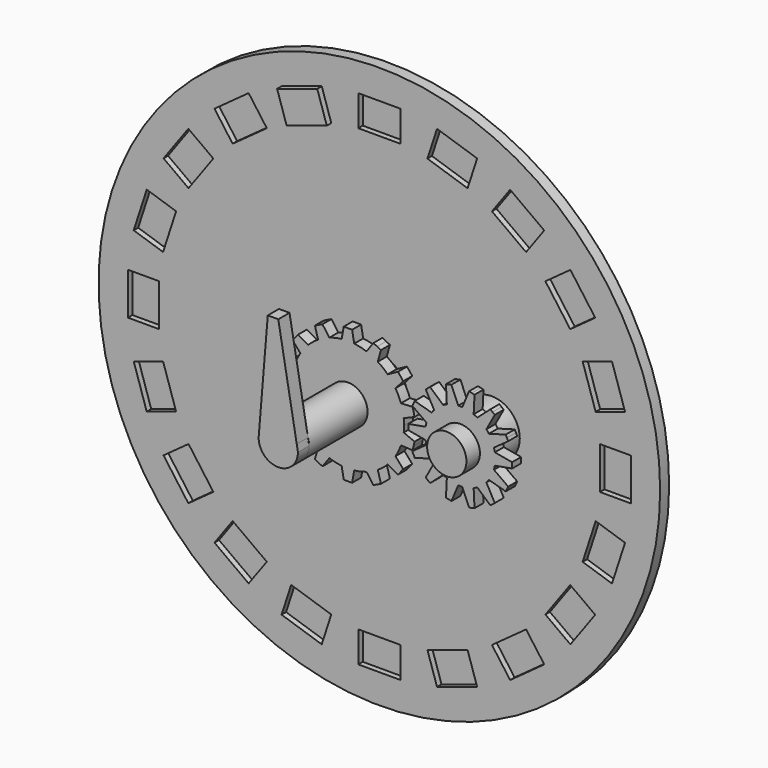
from build123d import *

# Parameters (mm, degrees)
F0_R      = 100
F1_DEPTH  = 4
F2_R      = 10
F2_R_2    = 7
F3_DEPTH  = 10
F4_DEPTH  = 40
F5_DEPTH  = 20
F7_DEPTH  = 4
F9_DEPTH  = 4
F10_W     = 15.0254992768
F10_H     = 11
F10_W_2   = 11
F10_H_2   = 15.0254992768
F11_DEPTH = 2
F12_DEPTH = 4
F14_DEPTH = 5


with BuildPart() as f1:
    # F0 (on Front) → F1 (new body)
    with BuildSketch(Plane.XZ):
        Circle(F0_R)
    extrude(amount=F1_DEPTH)

    # F2 (on face) → F3 (join)
    with BuildSketch(Plane.XZ.offset(4)):
        Circle(F2_R)
        Circle(F2_R_2, mode=Mode.SUBTRACT)
        with Locations((40, 0)):
            Circle(F2_R)
        with Locations((40, 0)):
            Circle(F2_R_2, mode=Mode.SUBTRACT)
    extrude(amount=F3_DEPTH)


with BuildPart() as f4:
    # F4 (new): a face of the model
    f4_faces = [f1.part.faces().sort_by_distance(p)[0] for p in [
        (0, -4, 0),
    ]]
    extrude(f4_faces, amount=F4_DEPTH)

    # F6 (on face) → F7 (join)
    with BuildSketch(Plane.XZ.offset(14)):
        with BuildLine():
            ThreePointArc((19.8728833209, -2.2513348298), (19.9681955421, -1.1274603281), (20, 0))
            ThreePointArc((20, 0), (19.9681955421, 1.1274603281), (19.8728833209, 2.2513348298))
            ThreePointArc((19.8728833209, 2.2513348298), (19.4985582436, 4.4504186791), (18.8816667615, 6.5941383294))
            ThreePointArc((18.8816667615, 6.5941383294), (18.019377358, 8.6776747824), (16.9280316136, 10.6509035152))
            ThreePointArc((16.9280316136, 10.6509035152), (15.6366296494, 12.4697960372), (14.1507045316, 14.1335615207))
            ThreePointArc((14.1507045316, 14.1335615207), (12.4697960372, 15.6366296494), (10.6303756366, 16.9409301346))
            ThreePointArc((10.6303756366, 16.9409301346), (8.6776747824, 18.019377358), (6.6170217222, 18.8736595161))
            ThreePointArc((6.6170217222, 18.8736595161), (4.4504186791, 19.4985582436), (2.2272433917, 19.875597774))
            ThreePointArc((2.2272433917, 19.875597774), (0, 20), (-2.2272433917, 19.875597774))
            ThreePointArc((-2.2272433917, 19.875597774), (-4.4504186791, 19.4985582436), (-6.6170217222, 18.8736595161))
            ThreePointArc((-6.6170217222, 18.8736595161), (-8.6776747824, 18.019377358), (-10.6303756366, 16.9409301346))
            ThreePointArc((-10.6303756366, 16.9409301346), (-12.4697960372, 15.6366296494), (-14.1507045316, 14.1335615207))
            ThreePointArc((-14.1507045316, 14.1335615207), (-15.6366296494, 12.4697960372), (-16.9280316136, 10.6509035152))
            ThreePointArc((-16.9280316136, 10.6509035152), (-18.019377358, 8.6776747824), (-18.8816667615, 6.5941383294))
            ThreePointArc((-18.8816667615, 6.5941383294), (-19.4985582436, 4.4504186791), (-19.8728833209, 2.2513348298))
            ThreePointArc((-19.8728833209, 2.2513348298), (-20, 0), (-19.8728833209, -2.2513348298))
            ThreePointArc((-19.8728833209, -2.2513348298), (-19.4985582436, -4.4504186791), (-18.8816667615, -6.5941383294))
            ThreePointArc((-18.8816667615, -6.5941383294), (-18.019377358, -8.6776747824), (-16.9280316136, -10.6509035152))
            ThreePointArc((-16.9280316136, -10.6509035152), (-15.6366296494, -12.4697960372), (-14.1507045316, -14.1335615207))
            ThreePointArc((-14.1507045316, -14.1335615207), (-12.4697960372, -15.6366296494), (-10.6303756366, -16.9409301346))
            ThreePointArc((-10.6303756366, -16.9409301346), (-8.6776747824, -18.019377358), (-6.6170217222, -18.8736595161))
            ThreePointArc((-6.6170217222, -18.8736595161), (-4.4504186791, -19.4985582436), (-2.2272433917, -19.875597774))
            ThreePointArc((-2.2272433917, -19.875597774), (0, -20), (2.2272433917, -19.875597774))
            ThreePointArc((2.2272433917, -19.875597774), (4.4504186791, -19.4985582436), (6.6170217222, -18.8736595161))
            ThreePointArc((6.6170217222, -18.8736595161), (8.6776747824, -18.019377358), (10.6303756366, -16.9409301346))
            ThreePointArc((10.6303756366, -16.9409301346), (12.4697960372, -15.6366296494), (14.1507045316, -14.1335615207))
            ThreePointArc((14.1507045316, -14.1335615207), (15.6366296494, -12.4697960372), (16.9280316136, -10.6509035152))
            ThreePointArc((16.9280316136, -10.6509035152), (18.019377358, -8.6776747824), (18.8816667615, -6.5941383294))
            ThreePointArc((18.8816667615, -6.5941383294), (19.4985582436, -4.4504186791), (19.8728833209, -2.2513348298))
        make_face()
        with BuildLine():
            ThreePointArc((18.8816667615, 6.5941383294), (19.4985582436, 4.4504186791), (19.8728833209, 2.2513348298))
            Line((19.8728833209, 2.2513348298), (23.7320512933, 3.8781105467))
            Line((23.7320512933, 3.8781105467), (23.3982698924, 5.340502415))
            Line((23.3982698924, 5.340502415), (23.0644884914, 6.8028942832))
            Line((23.0644884914, 6.8028942832), (18.8816667615, 6.5941383294))
        make_face()
        with BuildLine():
            Line((23.7320512933, -3.8781105467), (19.8728833209, -2.2513348298))
            ThreePointArc((19.8728833209, -2.2513348298), (19.4985582436, -4.4504186791), (18.8816667615, -6.5941383294))
            Line((18.8816667615, -6.5941383294), (23.0644884914, -6.8028942832))
            Line((23.0644884914, -6.8028942832), (23.3982698924, -5.340502415))
            Line((23.3982698924, -5.340502415), (23.7320512933, -3.8781105467))
        make_face()
        with BuildLine():
            ThreePointArc((14.1507045316, 14.1335615207), (15.6366296494, 12.4697960372), (16.9280316136, 10.6509035152))
            Line((16.9280316136, 10.6509035152), (19.699190282, 13.7910080209))
            Line((19.699190282, 13.7910080209), (18.7639555792, 14.9637552446))
            Line((18.7639555792, 14.9637552446), (17.8287208764, 16.1365024683))
            Line((17.8287208764, 16.1365024683), (14.1507045316, 14.1335615207))
        make_face()
        with BuildLine():
            Line((19.699190282, -13.7910080209), (16.9280316136, -10.6509035152))
            ThreePointArc((16.9280316136, -10.6509035152), (15.6366296494, -12.4697960372), (14.1507045316, -14.1335615207))
            Line((14.1507045316, -14.1335615207), (17.8287208764, -16.1365024683))
            Line((17.8287208764, -16.1365024683), (18.7639555792, -14.9637552446))
            Line((18.7639555792, -14.9637552446), (19.699190282, -13.7910080209))
        make_face()
        with BuildLine():
            ThreePointArc((6.6170217222, 18.8736595161), (8.6776747824, 18.019377358), (10.6303756366, 16.9409301346))
            Line((10.6303756366, 16.9409301346), (11.7646630407, 20.972427221))
            Line((11.7646630407, 20.972427221), (10.4132097388, 21.6232528297))
            Line((10.4132097388, 21.6232528297), (9.061756437, 22.2740784383))
            Line((9.061756437, 22.2740784383), (6.6170217222, 18.8736595161))
        make_face()
        with BuildLine():
            Line((11.7646630407, -20.972427221), (10.6303756366, -16.9409301346))
            ThreePointArc((10.6303756366, -16.9409301346), (8.6776747824, -18.019377358), (6.6170217222, -18.8736595161))
            Line((6.6170217222, -18.8736595161), (9.061756437, -22.2740784383))
            Line((9.061756437, -22.2740784383), (10.4132097388, -21.6232528297))
            Line((10.4132097388, -21.6232528297), (11.7646630407, -20.972427221))
        make_face()
        with BuildLine():
            ThreePointArc((-2.2272433917, 19.875597774), (0, 20), (2.2272433917, 19.875597774))
            Line((2.2272433917, 19.875597774), (1.5, 24))
            Line((1.5, 24), (0, 24))
            Line((0, 24), (-1.5, 24))
            Line((-1.5, 24), (-2.2272433917, 19.875597774))
        make_face()
        with BuildLine():
            Line((1.5, -24), (2.2272433917, -19.875597774))
            ThreePointArc((2.2272433917, -19.875597774), (0, -20), (-2.2272433917, -19.875597774))
            Line((-2.2272433917, -19.875597774), (-1.5, -24))
            Line((-1.5, -24), (0, -24))
            Line((0, -24), (1.5, -24))
        make_face()
        with BuildLine():
            ThreePointArc((-10.6303756366, 16.9409301346), (-8.6776747824, 18.019377358), (-6.6170217222, 18.8736595161))
            Line((-6.6170217222, 18.8736595161), (-9.061756437, 22.2740784383))
            Line((-9.061756437, 22.2740784383), (-10.4132097388, 21.6232528297))
            Line((-10.4132097388, 21.6232528297), (-11.7646630407, 20.972427221))
            Line((-11.7646630407, 20.972427221), (-10.6303756366, 16.9409301346))
        make_face()
        with BuildLine():
            Line((-9.061756437, -22.2740784383), (-6.6170217222, -18.8736595161))
            ThreePointArc((-6.6170217222, -18.8736595161), (-8.6776747824, -18.019377358), (-10.6303756366, -16.9409301346))
            Line((-10.6303756366, -16.9409301346), (-11.7646630407, -20.972427221))
            Line((-11.7646630407, -20.972427221), (-10.4132097388, -21.6232528297))
            Line((-10.4132097388, -21.6232528297), (-9.061756437, -22.2740784383))
        make_face()
        with BuildLine():
            ThreePointArc((-16.9280316136, 10.6509035152), (-15.6366296494, 12.4697960372), (-14.1507045316, 14.1335615207))
            Line((-14.1507045316, 14.1335615207), (-17.8287208764, 16.1365024683))
            Line((-17.8287208764, 16.1365024683), (-18.7639555792, 14.9637552446))
            Line((-18.7639555792, 14.9637552446), (-19.699190282, 13.7910080209))
            Line((-19.699190282, 13.7910080209), (-16.9280316136, 10.6509035152))
        make_face()
        with BuildLine():
            Line((-17.8287208764, -16.1365024683), (-14.1507045316, -14.1335615207))
            ThreePointArc((-14.1507045316, -14.1335615207), (-15.6366296494, -12.4697960372), (-16.9280316136, -10.6509035152))
            Line((-16.9280316136, -10.6509035152), (-19.699190282, -13.7910080209))
            Line((-19.699190282, -13.7910080209), (-18.7639555792, -14.9637552446))
            Line((-18.7639555792, -14.9637552446), (-17.8287208764, -16.1365024683))
        make_face()
        with BuildLine():
            ThreePointArc((-19.8728833209, 2.2513348298), (-19.4985582436, 4.4504186791), (-18.8816667615, 6.5941383294))
            Line((-18.8816667615, 6.5941383294), (-23.0644884914, 6.8028942832))
            Line((-23.0644884914, 6.8028942832), (-23.3982698924, 5.340502415))
            Line((-23.3982698924, 5.340502415), (-23.7320512933, 3.8781105467))
            Line((-23.7320512933, 3.8781105467), (-19.8728833209, 2.2513348298))
        make_face()
        with BuildLine():
            Line((-23.0644884914, -6.8028942832), (-18.8816667615, -6.5941383294))
            ThreePointArc((-18.8816667615, -6.5941383294), (-19.4985582436, -4.4504186791), (-19.8728833209, -2.2513348298))
            Line((-19.8728833209, -2.2513348298), (-23.7320512933, -3.8781105467))
            Line((-23.7320512933, -3.8781105467), (-23.3982698924, -5.340502415))
            Line((-23.3982698924, -5.340502415), (-23.0644884914, -6.8028942832))
        make_face()
    extrude(amount=F7_DEPTH)

    # F13 (on face) → F14 (join)
    with BuildSketch(Plane.XZ.offset(44)):
        with BuildLine():
            Line((-6.905075168, 1.1488850788), (-7, 0))
            ThreePointArc((-7, 0), (0, -7), (7, 0))
            Line((7, 0), (6.57125, 2.4121926618))
            ThreePointArc((6.57125, 2.4121926618), (-0.653334771, 6.9694442875), (-6.905075168, 1.1488850788))
        make_face()
        with BuildLine():
            Line((-3.7460629491, 39.382737335), (-6.905075168, 1.1488850788))
            ThreePointArc((-6.905075168, 1.1488850788), (-0.653334771, 6.9694442875), (6.57125, 2.4121926618))
            Line((6.57125, 2.4121926618), (0, 39.382737335))
            Line((0, 39.382737335), (-3.7460629491, 39.382737335))
        make_face()
    extrude(amount=F14_DEPTH)


with BuildPart() as f5:
    # F5 (new): a face of the model
    f5_faces = [f1.part.faces().sort_by_distance(p)[0] for p in [
        (40, -4, 0),
    ]]
    extrude(f5_faces, amount=F5_DEPTH)

    # F8 (on face) → F9 (join)
    with BuildSketch(Plane.XZ.offset(14)):
        with BuildLine():
            ThreePointArc((52.3250464347, -2.0840418379), (52.4561848179, -1.0456862737), (52.5, 0))
            ThreePointArc((52.5, 0), (52.4561848179, 1.0456862737), (52.3250464347, 2.0840418379))
            ThreePointArc((52.3250464347, 2.0840418379), (52.1865989023, 2.7815116745), (52.0087149982, 3.4699804165))
            ThreePointArc((52.0087149982, 3.4699804165), (51.2621108488, 5.423546739), (50.200251268, 7.2252940473))
            ThreePointArc((50.200251268, 7.2252940473), (49.7728935309, 7.7936225232), (49.3139102792, 8.3367304929))
            ThreePointArc((49.3139102792, 8.3367304929), (47.7936225232, 9.7728935309), (46.0551712398, 10.9354881581))
            ThreePointArc((46.0551712398, 10.9354881581), (45.423546739, 11.2621108488), (44.7743714017, 11.552288852))
            ThreePointArc((44.7743714017, 11.552288852), (42.7815116745, 12.1865989023), (40.7107902857, 12.4797747243))
            ThreePointArc((40.7107902857, 12.4797747243), (40, 12.5), (39.2892097143, 12.4797747243))
            ThreePointArc((39.2892097143, 12.4797747243), (37.2184883255, 12.1865989023), (35.2256285983, 11.552288852))
            ThreePointArc((35.2256285983, 11.552288852), (34.576453261, 11.2621108488), (33.9448287602, 10.9354881581))
            ThreePointArc((33.9448287602, 10.9354881581), (32.2063774768, 9.7728935309), (30.6860897208, 8.3367304929))
            ThreePointArc((30.6860897208, 8.3367304929), (30.2271064691, 7.7936225232), (29.799748732, 7.2252940473))
            ThreePointArc((29.799748732, 7.2252940473), (28.7378891512, 5.423546739), (27.9912850018, 3.4699804165))
            ThreePointArc((27.9912850018, 3.4699804165), (27.8134010977, 2.7815116745), (27.6749535653, 2.0840418379))
            ThreePointArc((27.6749535653, 2.0840418379), (27.5, 0), (27.6749535653, -2.0840418379))
            ThreePointArc((27.6749535653, -2.0840418379), (27.8134010977, -2.7815116745), (27.9912850018, -3.4699804165))
            ThreePointArc((27.9912850018, -3.4699804165), (28.7378891512, -5.423546739), (29.799748732, -7.2252940473))
            ThreePointArc((29.799748732, -7.2252940473), (30.2271064691, -7.7936225232), (30.6860897208, -8.3367304929))
            ThreePointArc((30.6860897208, -8.3367304929), (32.2063774768, -9.7728935309), (33.9448287602, -10.9354881581))
            ThreePointArc((33.9448287602, -10.9354881581), (34.576453261, -11.2621108488), (35.2256285983, -11.552288852))
            ThreePointArc((35.2256285983, -11.552288852), (37.2184883255, -12.1865989023), (39.2892097143, -12.4797747243))
            ThreePointArc((39.2892097143, -12.4797747243), (40, -12.5), (40.7107902857, -12.4797747243))
            ThreePointArc((40.7107902857, -12.4797747243), (42.7815116745, -12.1865989023), (44.7743714017, -11.552288852))
            ThreePointArc((44.7743714017, -11.552288852), (45.423546739, -11.2621108488), (46.0551712398, -10.9354881581))
            ThreePointArc((46.0551712398, -10.9354881581), (47.7936225232, -9.7728935309), (49.3139102792, -8.3367304929))
            ThreePointArc((49.3139102792, -8.3367304929), (49.7728935309, -7.7936225232), (50.200251268, -7.2252940473))
            ThreePointArc((50.200251268, -7.2252940473), (51.2621108488, -5.423546739), (52.0087149982, -3.4699804165))
            ThreePointArc((52.0087149982, -3.4699804165), (52.1865989023, -2.7815116745), (52.3250464347, -2.0840418379))
        make_face()
        with BuildLine():
            ThreePointArc((52.3250464347, 2.0840418379), (52.4561848179, 1.0456862737), (52.5, 0))
            ThreePointArc((52.5, 0), (52.4561848179, -1.0456862737), (52.3250464347, -2.0840418379))
            Line((52.3250464347, -2.0840418379), (58.4729532019, -1))
            Line((58.4729532019, -1), (58.4729532019, 0))
            Line((58.4729532019, 0), (58.4729532019, 1))
            Line((58.4729532019, 1), (52.3250464347, 2.0840418379))
        make_face()
        with BuildLine():
            ThreePointArc((50.200251268, 7.2252940473), (51.2621108488, 5.423546739), (52.0087149982, 3.4699804165))
            Line((52.0087149982, 3.4699804165), (57.0774394723, 7.1141451399))
            Line((57.0774394723, 7.1141451399), (56.6435557331, 8.0151140078))
            Line((56.6435557331, 8.0151140078), (56.209671994, 8.9160828757))
            Line((56.209671994, 8.9160828757), (50.200251268, 7.2252940473))
        make_face()
        with BuildLine():
            Line((57.0774394723, -7.1141451399), (52.0087149982, -3.4699804165))
            ThreePointArc((52.0087149982, -3.4699804165), (51.2621108488, -5.423546739), (50.200251268, -7.2252940473))
            Line((50.200251268, -7.2252940473), (56.209671994, -8.9160828757))
            Line((56.209671994, -8.9160828757), (56.6435557331, -8.0151140078))
            Line((56.6435557331, -8.0151140078), (57.0774394723, -7.1141451399))
        make_face()
        with BuildLine():
            ThreePointArc((46.0551712398, 10.9354881581), (47.7936225232, 9.7728935309), (49.3139102792, 8.3367304929))
            Line((49.3139102792, 8.3367304929), (52.2995294141, 13.8192465856))
            Line((52.2995294141, 13.8192465856), (51.5176979316, 14.4427363874))
            Line((51.5176979316, 14.4427363874), (50.7358664491, 15.0662261893))
            Line((50.7358664491, 15.0662261893), (46.0551712398, 10.9354881581))
        make_face()
        with BuildLine():
            Line((52.2995294141, -13.8192465856), (49.3139102792, -8.3367304929))
            ThreePointArc((49.3139102792, -8.3367304929), (47.7936225232, -9.7728935309), (46.0551712398, -10.9354881581))
            Line((46.0551712398, -10.9354881581), (50.7358664491, -15.0662261893))
            Line((50.7358664491, -15.0662261893), (51.5176979316, -14.4427363874))
            Line((51.5176979316, -14.4427363874), (52.2995294141, -13.8192465856))
        make_face()
        with BuildLine():
            ThreePointArc((40.7107902857, 12.4797747243), (42.7815116745, 12.1865989023), (44.7743714017, 11.552288852))
            Line((44.7743714017, 11.552288852), (45.0855467116, 17.787276763))
            Line((45.0855467116, 17.787276763), (44.1106187994, 18.009797697))
            Line((44.1106187994, 18.009797697), (43.1356908872, 18.2323186309))
            Line((43.1356908872, 18.2323186309), (40.7107902857, 12.4797747243))
        make_face()
        with BuildLine():
            Line((45.0855467116, -17.787276763), (44.7743714017, -11.552288852))
            ThreePointArc((44.7743714017, -11.552288852), (42.7815116745, -12.1865989023), (40.7107902857, -12.4797747243))
            Line((40.7107902857, -12.4797747243), (43.1356908872, -18.2323186309))
            Line((43.1356908872, -18.2323186309), (44.1106187994, -18.009797697))
            Line((44.1106187994, -18.009797697), (45.0855467116, -17.787276763))
        make_face()
        with BuildLine():
            ThreePointArc((35.2256285983, 11.552288852), (37.2184883255, 12.1865989023), (39.2892097143, 12.4797747243))
            Line((39.2892097143, 12.4797747243), (36.8643091128, 18.2323186309))
            Line((36.8643091128, 18.2323186309), (35.8893812006, 18.009797697))
            Line((35.8893812006, 18.009797697), (34.9144532884, 17.787276763))
            Line((34.9144532884, 17.787276763), (35.2256285983, 11.552288852))
        make_face()
        with BuildLine():
            Line((36.8643091128, -18.2323186309), (39.2892097143, -12.4797747243))
            ThreePointArc((39.2892097143, -12.4797747243), (37.2184883255, -12.1865989023), (35.2256285983, -11.552288852))
            Line((35.2256285983, -11.552288852), (34.9144532884, -17.787276763))
            Line((34.9144532884, -17.787276763), (35.8893812006, -18.009797697))
            Line((35.8893812006, -18.009797697), (36.8643091128, -18.2323186309))
        make_face()
        with BuildLine():
            ThreePointArc((30.6860897208, 8.3367304929), (32.2063774768, 9.7728935309), (33.9448287602, 10.9354881581))
            Line((33.9448287602, 10.9354881581), (29.2641335509, 15.0662261893))
            Line((29.2641335509, 15.0662261893), (28.4823020684, 14.4427363874))
            Line((28.4823020684, 14.4427363874), (27.7004705859, 13.8192465856))
            Line((27.7004705859, 13.8192465856), (30.6860897208, 8.3367304929))
        make_face()
        with BuildLine():
            Line((29.2641335509, -15.0662261893), (33.9448287602, -10.9354881581))
            ThreePointArc((33.9448287602, -10.9354881581), (32.2063774768, -9.7728935309), (30.6860897208, -8.3367304929))
            Line((30.6860897208, -8.3367304929), (27.7004705859, -13.8192465856))
            Line((27.7004705859, -13.8192465856), (28.4823020684, -14.4427363874))
            Line((28.4823020684, -14.4427363874), (29.2641335509, -15.0662261893))
        make_face()
        with BuildLine():
            ThreePointArc((27.9912850018, 3.4699804165), (28.7378891512, 5.423546739), (29.799748732, 7.2252940473))
            Line((29.799748732, 7.2252940473), (23.790328006, 8.9160828757))
            Line((23.790328006, 8.9160828757), (23.3564442669, 8.0151140078))
            Line((23.3564442669, 8.0151140078), (22.9225605277, 7.1141451399))
            Line((22.9225605277, 7.1141451399), (27.9912850018, 3.4699804165))
        make_face()
        with BuildLine():
            Line((23.790328006, -8.9160828757), (29.799748732, -7.2252940473))
            ThreePointArc((29.799748732, -7.2252940473), (28.7378891512, -5.423546739), (27.9912850018, -3.4699804165))
            Line((27.9912850018, -3.4699804165), (22.9225605277, -7.1141451399))
            Line((22.9225605277, -7.1141451399), (23.3564442669, -8.0151140078))
            Line((23.3564442669, -8.0151140078), (23.790328006, -8.9160828757))
        make_face()
        with BuildLine():
            ThreePointArc((27.6749535653, -2.0840418379), (27.5, 0), (27.6749535653, 2.0840418379))
            Line((27.6749535653, 2.0840418379), (21.5270467981, 1))
            Line((21.5270467981, 1), (21.5270467981, 0))
            Line((21.5270467981, 0), (21.5270467981, -1))
            Line((21.5270467981, -1), (27.6749535653, -2.0840418379))
        make_face()
    extrude(amount=F9_DEPTH)


with BuildPart() as f1_1:
    add(f1.part)

    # F10 (on face) → F11 (cut)
    with BuildSketch(Plane.XZ.offset(4)):
        with Locations((0, 84.0504131913)):
            Rectangle(F10_W, F10_H)
        Polygon((-17.1283630924, 77.027449636), (-20.5275500305, 87.4890713153), (-34.8176490283, 82.8459366898), (-31.4184620902, 72.3843150105), align=None)
        Polygon((-40.0928323034, 67.9645026286), (-46.5584700786, 76.8636895667), (-58.7143543425, 68.0319226835), (-52.2487165673, 59.1327357453), align=None)
        Polygon((-59.1327357453, 52.2487165673), (-68.0319226835, 58.7143543425), (-76.8636895667, 46.5584700786), (-67.9645026286, 40.0928323034), align=None)
        Polygon((-72.3843150105, 31.4184620902), (-82.8459366898, 34.8176490283), (-87.4890713153, 20.5275500305), (-77.027449636, 17.1283630924), align=None)
        with Locations((-84.0504131913, 0)):
            Rectangle(F10_W_2, F10_H_2)
        Polygon((-77.027449636, -17.1283630924), (-87.4890713153, -20.5275500305), (-82.8459366898, -34.8176490283), (-72.3843150105, -31.4184620902), align=None)
        Polygon((-67.9645026286, -40.0928323034), (-76.8636895667, -46.5584700786), (-68.0319226835, -58.7143543425), (-59.1327357453, -52.2487165673), align=None)
        Polygon((-52.2487165673, -59.1327357453), (-58.7143543425, -68.0319226835), (-46.5584700786, -76.8636895667), (-40.0928323034, -67.9645026286), align=None)
        Polygon((-31.4184620902, -72.3843150105), (-34.8176490283, -82.8459366898), (-20.5275500305, -87.4890713153), (-17.1283630924, -77.027449636), align=None)
        with Locations((0, -84.0504131913)):
            Rectangle(F10_W, F10_H)
        Polygon((17.1283630924, -77.027449636), (20.5275500305, -87.4890713153), (34.8176490283, -82.8459366898), (31.4184620902, -72.3843150105), align=None)
        Polygon((40.0928323034, -67.9645026286), (46.5584700786, -76.8636895667), (58.7143543425, -68.0319226835), (52.2487165673, -59.1327357453), align=None)
        Polygon((59.1327357453, -52.2487165673), (68.0319226835, -58.7143543425), (76.8636895667, -46.5584700786), (67.9645026286, -40.0928323034), align=None)
        Polygon((72.3843150105, -31.4184620902), (82.8459366898, -34.8176490283), (87.4890713153, -20.5275500305), (77.027449636, -17.1283630924), align=None)
        with Locations((84.0504131913, 0)):
            Rectangle(F10_W_2, F10_H_2)
        Polygon((77.027449636, 17.1283630924), (87.4890713153, 20.5275500305), (82.8459366898, 34.8176490283), (72.3843150105, 31.4184620902), align=None)
        Polygon((67.9645026286, 40.0928323034), (76.8636895667, 46.5584700786), (68.0319226835, 58.7143543425), (59.1327357453, 52.2487165673), align=None)
        Polygon((52.2487165673, 59.1327357453), (58.7143543425, 68.0319226835), (46.5584700786, 76.8636895667), (40.0928323034, 67.9645026286), align=None)
        Polygon((31.4184620902, 72.3843150105), (34.8176490283, 82.8459366898), (20.5275500305, 87.4890713153), (17.1283630924, 77.027449636), align=None)
    extrude(amount=-F11_DEPTH, mode=Mode.SUBTRACT)


with BuildPart() as f12:
    # F12 (new): a face of the model
    f12_faces = [f1_1.part.faces().sort_by_distance(p)[0] for p in [
        (-25.9730060604, -2, 79.9366931629),
    ]]
    extrude(f12_faces, amount=F12_DEPTH)


solid = Compound([f4.part, f5.part, f1_1.part, f12.part])
